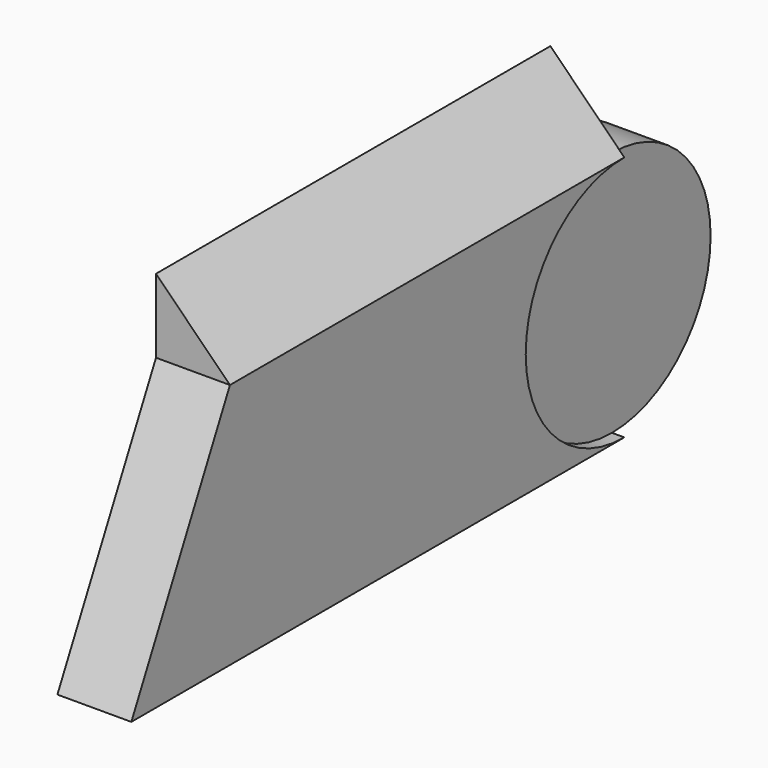
from build123d import *

# Parameters (mm, degrees)
F1_DEPTH = 15.24
F2_DEPTH = 12.7
F3_DEPTH = 15.24
F5_DEPTH = 101.6


# Not quite as in the source:
# - a feature names something its author has since deleted; it is built from what else it names


with BuildPart() as f1:
    # F0 (on Right) → F1 (new body)
    with BuildSketch(Plane.YZ):
        with BuildLine():
            ThreePointArc((37.1756509936, -4.7328671039), (19.2151387515, 2.7066206539), (11.7756509936, 20.6671328961))
            Line((11.7756509936, 20.6671328961), (-77.1243490064, 20.6671328961))
            Line((-77.1243490064, 20.6671328961), (-89.8243490064, -4.7328671039))
            Line((-89.8243490064, -4.7328671039), (37.1756509936, -4.7328671039))
        make_face()
        with BuildLine():
            Line((-77.1243490064, 20.6671328961), (11.7756509936, 20.6671328961))
            ThreePointArc((11.7756509936, 20.6671328961), (19.2151387515, 38.6276451382), (37.1756509936, 46.0671328961))
            Line((37.1756509936, 46.0671328961), (-64.4243490064, 46.0671328961))
            Line((-64.4243490064, 46.0671328961), (-77.1243490064, 20.6671328961))
        make_face()
    extrude(amount=F1_DEPTH)

    # F0 (on Right) → F2 (join)
    with BuildSketch(Plane.YZ):
        with BuildLine():
            Line((11.7756509936, 20.6671328961), (62.5756509936, 20.6671328961))
            ThreePointArc((62.5756509936, 20.6671328961), (55.1361632357, 38.6276451382), (37.1756509936, 46.0671328961))
            ThreePointArc((37.1756509936, 46.0671328961), (19.2151387515, 38.6276451382), (11.7756509936, 20.6671328961))
        make_face()
        with BuildLine():
            ThreePointArc((37.1756509936, -4.7328671039), (55.1361632357, 2.7066206539), (62.5756509936, 20.6671328961))
            Line((62.5756509936, 20.6671328961), (11.7756509936, 20.6671328961))
            ThreePointArc((11.7756509936, 20.6671328961), (19.2151387515, 2.7066206539), (37.1756509936, -4.7328671039))
        make_face()
    extrude(amount=F2_DEPTH)

    # F3 (add): a face of the model
    f3_faces = [f1.faces().sort_by_distance(p)[0] for p in [
        (7.62, -13.6243490064, 46.0671328961),
    ]]
    extrude(f3_faces, amount=F3_DEPTH)

    # F4 (on face) → F5 (cut)
    with BuildSketch(Plane.XZ.offset(64.4243490064)):
        Polygon((15.24, 61.3071328961), (0, 61.3071328961), (15.24, 46.0671328961), align=None)
    extrude(amount=-F5_DEPTH, mode=Mode.SUBTRACT)


solid = f1.part
